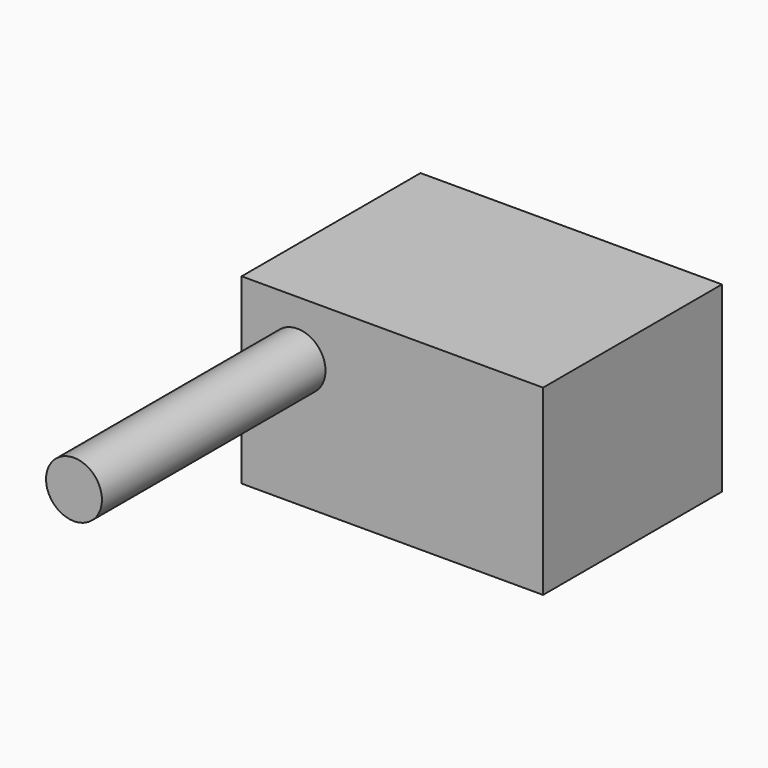
from build123d import *

# Parameters (mm, degrees)
F0_W     = 26.9646756351
F0_H     = 16.3272283971
F1_DEPTH = 20
F2_R     = 2.5
F3_DEPTH = 25


# Not quite as in the source:
# - the program builds the solid bodies; features that only make, move or delete a surface that nothing else refers to are left out


with BuildPart() as f1:
    # F0 (on Front) → F1 (new body)
    with BuildSketch(Plane.XZ):
        with Locations((-55.2899483591, 52.4450521916)):
            Rectangle(F0_W, F0_H)
    extrude(amount=F1_DEPTH)


with BuildPart() as f3:
    # F2 (on face) → F3 (new body)
    with BuildSketch(Plane.XZ.offset(20)):
        with Locations((-63.7722861767, 55.6086663902)):
            Circle(F2_R)
    extrude(amount=F3_DEPTH)


solid = Compound([f1.part, f3.part])
